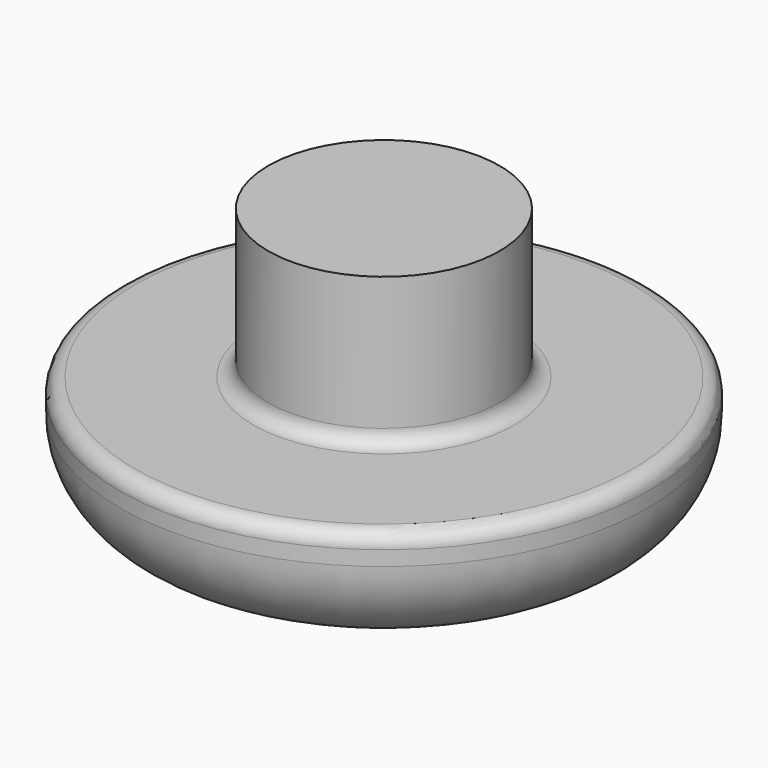
from build123d import *

# Parameters (mm, degrees)
F2_R = 0.5
F3_R = 3


with BuildPart() as f1:
    # F0 (on Front) → F1 (revolve)
    with BuildSketch(Plane.XZ):
        Polygon((-6.6499997675, -9.3892063797), (-6.6499997675, -14.3892063797), (-11.6499997675, -14.3892063797), (-11.6499997675, -18.3892063797), (-2.7499997675, -18.3892063797), (-2.7499997675, -9.3892063797), align=None)
    revolve(axis=Axis((-2.7499997675, 0, -13.8892063797), (0, 0, -1)))

    # F2
    f2_edges = [f1.edges().sort_by_distance(p)[0] for p in [
        (1.15, 0, -14.389206),
        (6.15, 0, -14.389206),
    ]]
    fillet(f2_edges, radius=F2_R)

    # F3
    f3_edges = [f1.edges().sort_by_distance(p)[0] for p in [
        (6.15, 0, -18.389206),
    ]]
    fillet(f3_edges, radius=F3_R)


solid = f1.part
